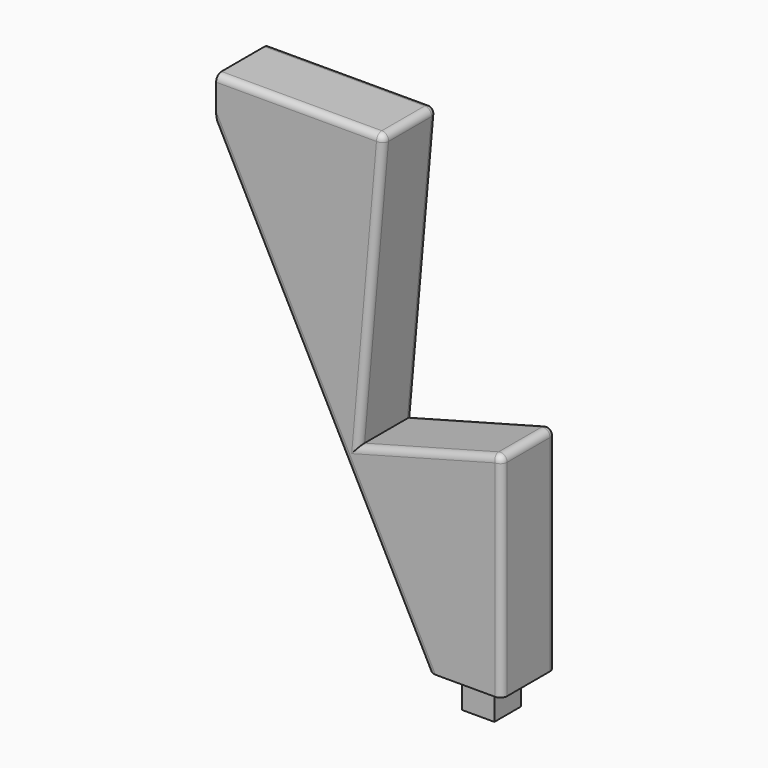
from build123d import *

# Parameters (mm, degrees)
F1_DEPTH      = 10
F3_W          = 4.8
F3_H          = 5
F4_DEPTH      = 5
F5_W          = 3
F5_H          = 3
F6_DEPTH      = 2.5
F7_R          = 1
F8_R          = 1
F9_R          = 1
F10_R         = 1
F11_R         = 1
F12_T1_DEPTH  = 33.1967746272
F12_T3_DEPTH  = 8
F12_T8_DEPTH  = 1
F12_T14_DEPTH = 1
F13_T1_DEPTH  = 26.4086914989
F13_T3_DEPTH  = 8
F13_T8_DEPTH  = 1
F13_T14_DEPTH = 1


# Not quite as in the source:
# - a fillet or chamfer that OpenCascade refuses, or shapes differently, is made with other operations: its cross-section is extruded or revolved along the edge and cut away or added


with BuildPart() as f1:
    # F0 (on Front) → F1 (new body)
    with BuildSketch(Plane.XZ):
        Polygon((25, 0), (0, 0), (0, -7), (31.589826983, -68.1461583276), (42.589826983, -68.1461583276), (42.589826983, -36.1461583276), (21.3394588046, -41.8401773199), align=None)
    extrude(amount=F1_DEPTH)

    # F3 (on face) → F4 (join)
    with BuildSketch(Plane(origin=(0, 0, -68.1461583276), x_dir=(1, 0, 0), z_dir=(0, 0, -1))):
        with Locations((37.089826983, 5)):
            Rectangle(F3_W, F3_H)
    extrude(amount=F4_DEPTH)

    # F5 (on face) → F6 (cut)
    with BuildSketch(Plane(origin=(0, 0, 0), x_dir=(0, -1, 0), z_dir=(-1, 0, 0))):
        with Locations((5, -3.5)):
            Rectangle(F5_W, F5_H)
    extrude(amount=-F6_DEPTH, mode=Mode.SUBTRACT)

    # F7
    f7_edges = [f1.edges().sort_by_distance(p)[0] for p in [
        (23.169729, -10, -20.920089),
    ]]
    fillet(f7_edges, radius=F7_R)

    # F8
    f8_edges = [f1.edges().sort_by_distance(p)[0] for p in [
        (23.169729, 0, -20.920089),
    ]]
    fillet(f8_edges, radius=F8_R)

    # F9
    f9_edges = [f1.edges().sort_by_distance(p)[0] for p in [
        (15.794913, 0, -37.573079),
        (15.794913, -10, -37.573079),
    ]]
    fillet(f9_edges, radius=F9_R)

    # F10
    f10_edges = [f1.edges().sort_by_distance(p)[0] for p in [
        (31.964643, 0, -38.993168),
    ]]
    fillet(f10_edges, radius=F10_R)

    # F11
    f11_edges = [f1.edges().sort_by_distance(p)[0] for p in [
        (31.964643, -10, -38.993168),
    ]]
    fillet(f11_edges, radius=F11_R)

    # F12: fillet of radius 1 on 1 edges, made by hand

    # F12_s2 → F12_t1 (cut)
    with BuildSketch(Plane.XY.offset(-70.6461583276)):
        with BuildLine():
            ThreePointArc((42.589826983, -1), (42.2969337641, -0.2928932188), (41.589826983, 0))
            Line((41.589826983, 0), (42.589826983, 0))
            Line((42.589826983, 0), (42.589826983, -1))
        make_face()
        with BuildLine():
            ThreePointArc((42.589826983, -9), (42.2969337641, -9.7071067812), (41.589826983, -10))
            Line((41.589826983, -10), (42.589826983, -10))
            Line((42.589826983, -10), (42.589826983, -9))
        make_face()
    extrude(amount=F12_T1_DEPTH, mode=Mode.SUBTRACT)

    # F12_s4 → F12_t3 (cut)
    with BuildSketch(Plane.XZ.offset(1)):
        with BuildLine():
            ThreePointArc((42.589826983, -37.4493837004), (42.198588412, -36.6560303601), (41.3310079379, -36.4834578742))
            Line((41.3310079379, -36.4834578742), (42.589826983, -36.1461583276))
            Line((42.589826983, -36.1461583276), (42.589826983, -37.4493837004))
        make_face()
    extrude(amount=F12_T3_DEPTH, mode=Mode.SUBTRACT)


with BuildPart() as f12_tool6:
    # F12_s7 → F12_t8 (new body)
    with BuildSketch(Plane.XZ.offset(1)):
        Polygon((41.589826983, -37.4493837004), (42.589826983, -37.4493837004), (42.589826983, -36.1461583276), (41.3310079379, -36.4834578742), align=None)
    extrude(amount=-F12_T8_DEPTH)

    # F12_s9 → F12_t10 (revolve, cut)
    with BuildSketch(Plane(origin=(41.589826983, -1, -37.4493837004), x_dir=(-0.608761429, 0, -0.7933533403), z_dir=(0.7933533403, 0, -0.608761429))):
        with BuildLine():
            ThreePointArc((0, -1), (1, 0), (0, 1))
            Line((0, 1), (0, -1))
        make_face()
    revolve(axis=Axis((41.589826983, -1, -37.4493837004), (0, 1, 0)), mode=Mode.SUBTRACT)


with BuildPart() as f1_1:
    add(f1.part)

    # F12_t5: cut F12_tool6
    add(f12_tool6.part, mode=Mode.SUBTRACT)


with BuildPart() as f12_tool12:
    # F12_s13 → F12_t14 (new body)
    with BuildSketch(Plane.XZ.offset(9)):
        Polygon((41.589826983, -37.4493837004), (42.589826983, -37.4493837004), (42.589826983, -36.1461583276), (41.3310079379, -36.4834578742), align=None)
    extrude(amount=F12_T14_DEPTH)

    # F12_s15 → F12_t16 (revolve, cut)
    with BuildSketch(Plane(origin=(41.589826983, -9, -37.4493837004), x_dir=(-0.608761429, 0, -0.7933533403), z_dir=(-0.7933533403, 0, 0.608761429))):
        with BuildLine():
            ThreePointArc((0, -1), (1, 0), (0, 1))
            Line((0, 1), (0, -1))
        make_face()
    revolve(axis=Axis((41.589826983, -9, -37.4493837004), (0, -1, 0)), mode=Mode.SUBTRACT)


with BuildPart() as f1_2:
    add(f1_1.part)

    # F12_t11: cut F12_tool12
    add(f12_tool12.part, mode=Mode.SUBTRACT)

    # F13: fillet of radius 1 on 3 edges, made by hand

    # F13_s2 → F13_t1 (cut)
    with BuildSketch(Plane.YZ.offset(-2.5)):
        with BuildLine():
            ThreePointArc((-10, -1), (-9.7071067812, -0.2928932188), (-9, 0))
            Line((-9, 0), (-10, 0))
            Line((-10, 0), (-10, -1))
        make_face()
        with BuildLine():
            ThreePointArc((-1, 0), (-0.2928932188, -0.2928932188), (0, -1))
            Line((0, -1), (0, 0))
            Line((0, 0), (-1, 0))
        make_face()
    extrude(amount=F13_T1_DEPTH, mode=Mode.SUBTRACT)

    # F13_s4 → F13_t3 (cut)
    with BuildSketch(Plane.XZ.offset(1)):
        with BuildLine():
            ThreePointArc((24.904886197, -1.0871557427), (24.6459688357, -0.3244097924), (23.9086914989, 0))
            Line((23.9086914989, 0), (25, 0))
            Line((25, 0), (24.904886197, -1.0871557427))
        make_face()
    extrude(amount=F13_T3_DEPTH, mode=Mode.SUBTRACT)


with BuildPart() as f13_tool6:
    # F13_s7 → F13_t8 (new body)
    with BuildSketch(Plane.XZ.offset(1)):
        Polygon((23.9086914989, -1), (24.904886197, -1.0871557427), (25, 0), (23.9086914989, 0), align=None)
    extrude(amount=-F13_T8_DEPTH)

    # F13_s9 → F13_t10 (revolve, cut)
    with BuildSketch(Plane(origin=(23.9086914989, -1, -1), x_dir=(-0.7372773368, 0, -0.6755902076), z_dir=(0.6755902076, 0, -0.7372773368))):
        with BuildLine():
            ThreePointArc((0, -1), (1, 0), (0, 1))
            Line((0, 1), (0, -1))
        make_face()
    revolve(axis=Axis((23.9086914989, -1, -1), (0, 1, 0)), mode=Mode.SUBTRACT)


with BuildPart() as f1_3:
    add(f1_2.part)

    # F13_t5: cut F13_tool6
    add(f13_tool6.part, mode=Mode.SUBTRACT)


with BuildPart() as f13_tool12:
    # F13_s13 → F13_t14 (new body)
    with BuildSketch(Plane.XZ.offset(9)):
        Polygon((23.9086914989, -1), (24.904886197, -1.0871557427), (25, 0), (23.9086914989, 0), align=None)
    extrude(amount=F13_T14_DEPTH)

    # F13_s15 → F13_t16 (revolve, cut)
    with BuildSketch(Plane(origin=(23.9086914989, -9, -1), x_dir=(-0.7372773368, 0, -0.6755902076), z_dir=(-0.6755902076, 0, 0.7372773368))):
        with BuildLine():
            ThreePointArc((0, -1), (1, 0), (0, 1))
            Line((0, 1), (0, -1))
        make_face()
    revolve(axis=Axis((23.9086914989, -9, -1), (0, -1, 0)), mode=Mode.SUBTRACT)


with BuildPart() as f1_4:
    add(f1_3.part)

    # F13_t11: cut F13_tool12
    add(f13_tool12.part, mode=Mode.SUBTRACT)


solid = f1_4.part
